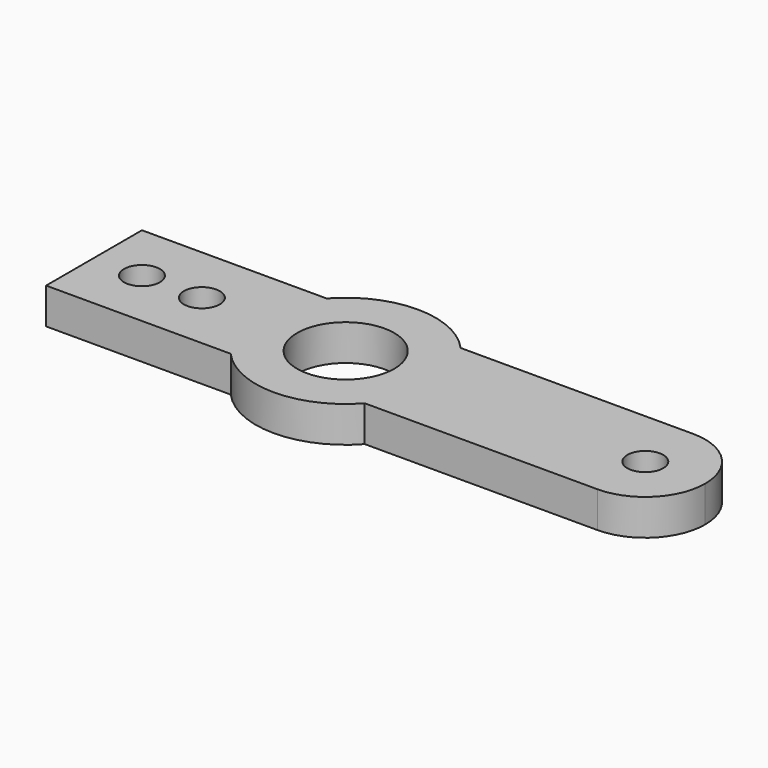
from build123d import *

# Parameters (mm, degrees)
F0_R     = 1.5
F0_R_2   = 4.05
F1_DEPTH = 3
F2_W     = 10
F2_H     = 3
F3_DEPTH = 9
F4_R     = 1.5
F5_DEPTH = 25
F6_R     = 4.99999


# Not quite as in the source:
# - a fillet or chamfer is up to 0.001 mm smaller than in the source, because OpenCascade refuses the exact size


with BuildPart() as f1:
    # F0 (on Top) → F1 (new body)
    with BuildSketch(Plane.XY):
        Polygon((21, -5), (21, 5), (5.5901699437, 5), (-5.5901699437, 5), (-21, 5), (-21, -5), (-5.5901699437, -5), (5.5901699437, -5), align=None)
        with Locations((-17, 0)):
            Circle(F0_R, mode=Mode.SUBTRACT)
        with Locations((-12, 0)):
            Circle(F0_R, mode=Mode.SUBTRACT)
        Circle(F0_R_2, mode=Mode.SUBTRACT)
        with BuildLine():
            Line((-5.5901699437, 5), (5.5901699437, 5))
            ThreePointArc((5.5901699437, 5), (0, 7.5), (-5.5901699437, 5))
        make_face()
        with BuildLine():
            ThreePointArc((-5.5901699437, -5), (0, -7.5), (5.5901699437, -5))
            Line((5.5901699437, -5), (-5.5901699437, -5))
        make_face()
    extrude(amount=F1_DEPTH)

    # F2 (on face) → F3 (join)
    with BuildSketch(Plane.YZ.offset(21)):
        with Locations((0, 1.5)):
            Rectangle(F2_W, F2_H)
    extrude(amount=F3_DEPTH)

    # F4 (on face) → F5 (cut)
    with BuildSketch(Plane(origin=(0, 0, 0), x_dir=(1, 0, 0), z_dir=(0, 0, -1))):
        with Locations((25, 0)):
            Circle(F4_R)
    extrude(amount=-F5_DEPTH, mode=Mode.SUBTRACT)

    # F6 (radius 5 in the source; OpenCascade refuses exactly that, so slightly less here)
    f6_edges = [f1.edges().sort_by_distance(p)[0] for p in [
        (30, -5, 1.5),
        (30, 5, 1.5),
    ]]
    fillet(f6_edges, radius=F6_R)


solid = f1.part
